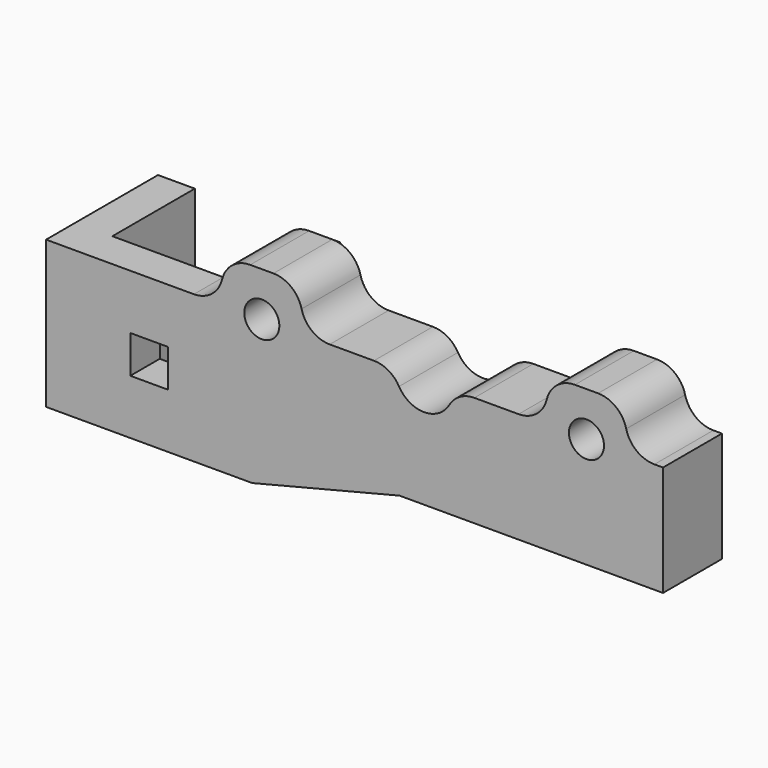
from build123d import *

# Parameters (mm, degrees)
F1_DEPTH      = 12.7
F2_R          = 3.25
F3_DEPTH      = 24.131
F4_W          = 6.5
F4_H          = 6.5
F5_DEPTH      = 7.62
F6_W          = 70.85
F6_H          = 12.7
F7_DEPTH      = 19.05
F9_DEPTH      = 6.35
F10_W         = 14
F10_H         = 12.7
F11_DEPTH     = 7.62
F12_R         = 5
F13_R         = 3.025
F14_DEPTH     = 24.131
F15_R         = 5
F16_DEPTH     = 24.131
F17_R         = 5
F19_DEPTH     = 4
F20_T1_DEPTH  = 12.7
F20_T6_DEPTH  = 12.7
F20_T12_DEPTH = 12.7
F20_T18_DEPTH = 12.7
F20_T21_DEPTH = 31.0012701892
F22_DEPTH     = 12


# Not quite as in the source:
# - a fillet or chamfer that OpenCascade refuses, or shapes differently, is made with other operations: its cross-section is extruded or revolved along the edge and cut away or added


with BuildPart() as f1:
    # F0 (on Top) → F1 (new body, symmetric)
    with BuildSketch(Plane.XY):
        Polygon((11.43, 8.001), (11.43, -9.779), (4.826, -9.779), (-7.366, -9.779), (-11.43, -9.779), (-11.43, 8.001), (-17.78, 8.001), (-17.78, -16.129), (17.78, -16.129), (17.78, 8.001), align=None)
    extrude(amount=F1_DEPTH, both=True)

    # F2 (on face) → F3 (cut, through all)
    with BuildSketch(Plane.XZ.offset(16.129)):
        Circle(F2_R)
    extrude(amount=-F3_DEPTH, mode=Mode.SUBTRACT)

    # F4 (on face) → F5 (cut)
    with BuildSketch(Plane.XZ.offset(16.129)):
        Rectangle(F4_W, F4_H)
    extrude(amount=-F5_DEPTH, mode=Mode.SUBTRACT)

    # F6 (on face) → F7 (join)
    with BuildSketch(Plane.XY.offset(12.7)):
        with Locations((53.205, -9.779)):
            Rectangle(F6_W, F6_H)
    extrude(amount=-F7_DEPTH)

    # F8 (on face) → F9 (join)
    with BuildSketch(Plane.XZ.offset(16.129)):
        Polygon((17.78, -6.35), (17.78, -12.7), (43.18, -6.35), align=None)
    extrude(amount=-F9_DEPTH)

    # F10 (on face) → F11 (join)
    with BuildSketch(Plane.XY.offset(12.7)):
        with Locations((19.43, -9.779)):
            Rectangle(F10_W, F10_H)
        with Locations((75.43, -9.779)):
            Rectangle(F10_W, F10_H)
    extrude(amount=F11_DEPTH)

    # F12
    f12_edges = [f1.edges().sort_by_distance(p)[0] for p in [
        (26.43, -9.779, 20.32),
        (12.43, -9.779, 20.32),
        (68.43, -9.779, 20.32),
        (82.43, -9.779, 20.32),
    ]]
    fillet(f12_edges, radius=F12_R)

    # F13 (on face) → F14 (cut, through all)
    with BuildSketch(Plane.XZ.offset(16.129)):
        with Locations((19.43, 12.7)):
            Circle(F13_R)
        with Locations((75.43, 12.7)):
            Circle(F13_R)
    extrude(amount=-F14_DEPTH, mode=Mode.SUBTRACT)

    # F15 (on face) → F16 (cut, through all)
    with BuildSketch(Plane.XZ.offset(16.129)):
        with Locations((47.43, 12.7)):
            Circle(F15_R)
    extrude(amount=-F16_DEPTH, mode=Mode.SUBTRACT)

    # F17
    f17_edges = [f1.edges().sort_by_distance(p)[0] for p in [
        (42.43, -9.779, 12.7),
    ]]
    fillet(f17_edges, radius=F17_R)

    # F18 (on face) → F19 (cut)
    with BuildSketch(Plane(origin=(0, -3.429, 0), x_dir=(-1, 0, 0), z_dir=(0, 1, 0))):
        Polygon((-69.6564973081, 12.7), (-72.5432486541, 17.7), (-78.3167513459, 17.7), (-81.2035026919, 12.7), (-78.3167513459, 7.7), (-72.5432486541, 7.7), align=None)
        Polygon((-25.2035026919, 12.7), (-22.3167513459, 7.7), (-16.5432486541, 7.7), (-13.6564973081, 12.7), (-16.5432486541, 17.7), (-22.3167513459, 17.7), align=None)
    extrude(amount=-F19_DEPTH, mode=Mode.SUBTRACT)

    # F20: fillet of radius 5 on 5 edges, made by hand

    # F20_s2 → F20_t1 (join)
    with BuildSketch(Plane.XZ.offset(3.429)):
        with BuildLine():
            ThreePointArc((82.2863257716, 16.51), (84.0563916708, 13.7661723474), (87.1426515432, 12.7))
            Line((87.1426515432, 12.7), (87.1426515432, 12.2))
            Line((87.1426515432, 12.2), (82.43, 12.2))
            Line((82.43, 12.2), (81.93, 12.7))
            ThreePointArc((81.93, 12.7), (81.93, 15.32), (81.8006931944, 16.391))
            Line((81.8006931944, 16.391), (82.2863257716, 16.51))
        make_face()
        with BuildLine():
            ThreePointArc((63.7173484568, 12.7), (66.8036083292, 13.7661723474), (68.5736742284, 16.51))
            Line((68.5736742284, 16.51), (69.0593068056, 16.391))
            ThreePointArc((69.0593068056, 16.391), (68.93, 15.32), (68.93, 12.7))
            Line((68.93, 12.7), (68.43, 12.2))
            Line((68.43, 12.2), (63.7173484568, 12.2))
            Line((63.7173484568, 12.2), (63.7173484568, 12.7))
        make_face()
        with BuildLine():
            ThreePointArc((31.1426515432, 12.7), (28.0563916708, 13.7661723474), (26.2863257716, 16.51))
            Line((26.2863257716, 16.51), (25.8006931944, 16.391))
            ThreePointArc((25.8006931944, 16.391), (25.93, 15.32), (25.93, 12.7))
            Line((25.93, 12.7), (26.43, 12.2))
            Line((26.43, 12.2), (31.1426515432, 12.2))
            Line((31.1426515432, 12.2), (31.1426515432, 12.7))
        make_face()
    extrude(amount=F20_T1_DEPTH)


with BuildPart() as f20_tool4:
    # F20_s5 → F20_t6 (new body)
    with BuildSketch(Plane.XZ.offset(3.429)):
        with BuildLine():
            ThreePointArc((12.5736742284, 16.51), (10.8036083292, 13.7661723474), (7.7173484568, 12.7))
            Line((7.7173484568, 12.7), (7.7173484568, 12.2))
            Line((7.7173484568, 12.2), (12.43, 12.2))
            Line((12.43, 12.2), (12.93, 12.7))
            ThreePointArc((12.93, 12.7), (12.93, 15.32), (13.0593068056, 16.391))
            Line((13.0593068056, 16.391), (12.5736742284, 16.51))
        make_face()
    extrude(amount=F20_T6_DEPTH)

    split(bisect_by=Plane.XZ.offset(9.779), keep=Keep.BOTTOM)

    split(bisect_by=Plane.YZ.offset(11.43), keep=Keep.TOP)


with BuildPart() as f1_1:
    add(f1.part)

    # F20_t3: union F20_tool4
    add(f20_tool4.part)


with BuildPart() as f20_tool10:
    # F20_s11 → F20_t12 (new body)
    with BuildSketch(Plane.XZ.offset(3.429)):
        with BuildLine():
            ThreePointArc((12.5736742284, 16.51), (10.8036083292, 13.7661723474), (7.7173484568, 12.7))
            Line((7.7173484568, 12.7), (7.7173484568, 12.2))
            Line((7.7173484568, 12.2), (12.43, 12.2))
            Line((12.43, 12.2), (12.93, 12.7))
            ThreePointArc((12.93, 12.7), (12.93, 15.32), (13.0593068056, 16.391))
            Line((13.0593068056, 16.391), (12.5736742284, 16.51))
        make_face()
    extrude(amount=F20_T12_DEPTH)

    split(bisect_by=Plane.XZ.offset(9.779), keep=Keep.TOP)

    split(bisect_by=Plane.YZ.offset(11.43), keep=Keep.TOP)


with BuildPart() as f1_2:
    add(f1_1.part)

    # F20_t9: union F20_tool10
    add(f20_tool10.part)


with BuildPart() as f20_tool16:
    # F20_s17 → F20_t18 (new body)
    with BuildSketch(Plane.XZ.offset(3.429)):
        with BuildLine():
            ThreePointArc((12.5736742284, 16.51), (10.8036083292, 13.7661723474), (7.7173484568, 12.7))
            Line((7.7173484568, 12.7), (7.7173484568, 12.2))
            Line((7.7173484568, 12.2), (12.43, 12.2))
            Line((12.43, 12.2), (12.93, 12.7))
            ThreePointArc((12.93, 12.7), (12.93, 15.32), (13.0593068056, 16.391))
            Line((13.0593068056, 16.391), (12.5736742284, 16.51))
        make_face()
    extrude(amount=F20_T18_DEPTH)

    split(bisect_by=Plane.XZ.offset(9.779), keep=Keep.TOP)

    split(bisect_by=Plane.YZ.offset(11.43), keep=Keep.BOTTOM)


with BuildPart() as f1_3:
    add(f1_2.part)

    # F20_t15: union F20_tool16
    add(f20_tool16.part)

    # F20_s22 → F20_t21 (cut)
    with BuildSketch(Plane.XZ.offset(-5.7216350946)):
        with BuildLine():
            ThreePointArc((51.7601270189, 10.2), (53.5902540378, 12.0301270189), (56.0902540378, 12.7))
            Line((56.0902540378, 12.7), (52.43, 12.7))
            ThreePointArc((52.43, 12.7), (52.2596291314, 11.4059047745), (51.7601270189, 10.2))
        make_face()
    extrude(amount=F20_T21_DEPTH, mode=Mode.SUBTRACT)

    # F21 (on face) → F22 (cut)
    with BuildSketch(Plane(origin=(0, 8.001, 0), x_dir=(-1, 0, 0), z_dir=(0, 1, 0))):
        Polygon((-22.3456188594, 7.65), (-16.5143811406, 7.65), (-13.5987622812, 12.7), (-16.5143811406, 17.75), (-22.3456188594, 17.75), (-25.2612377188, 12.7), align=None)
    extrude(amount=-F22_DEPTH, mode=Mode.SUBTRACT)


solid = f1_3.part
